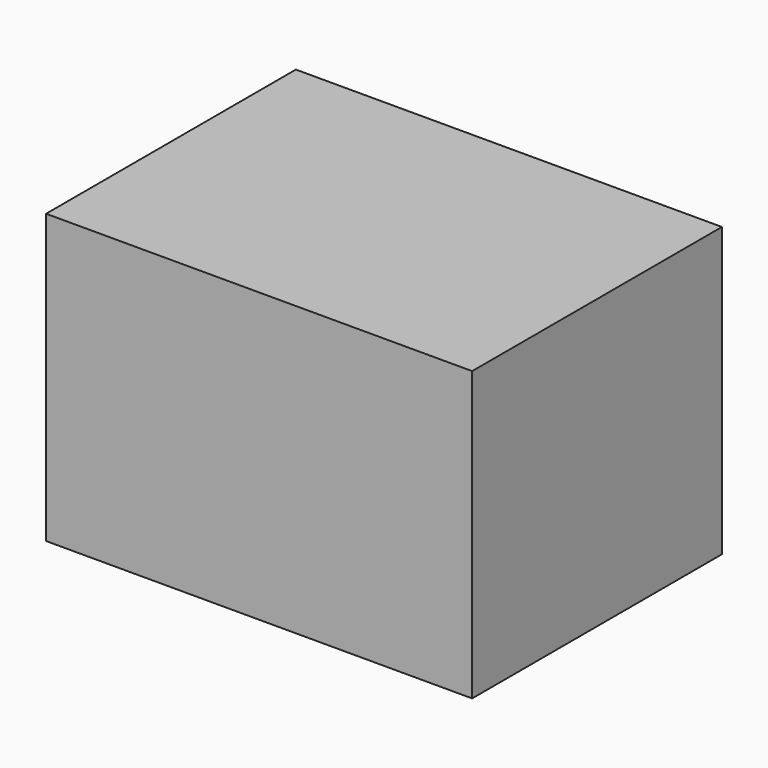
from build123d import *

# Parameters (mm, degrees)
F0_W     = 143.4638276696
F0_H     = 105.1291488111
F1_DEPTH = 97.028


# Not quite as in the source:
# - a feature of the source that left no trace in its solid (it failed there, or was rolled back) is left out


with BuildPart() as f1:
    # F0 (on Top) → F1 (new body)
    with BuildSketch(Plane.XY):
        with Locations((-35.3590212762, 17.8365651518)):
            Rectangle(F0_W, F0_H)
    extrude(amount=F1_DEPTH)


solid = f1.part
